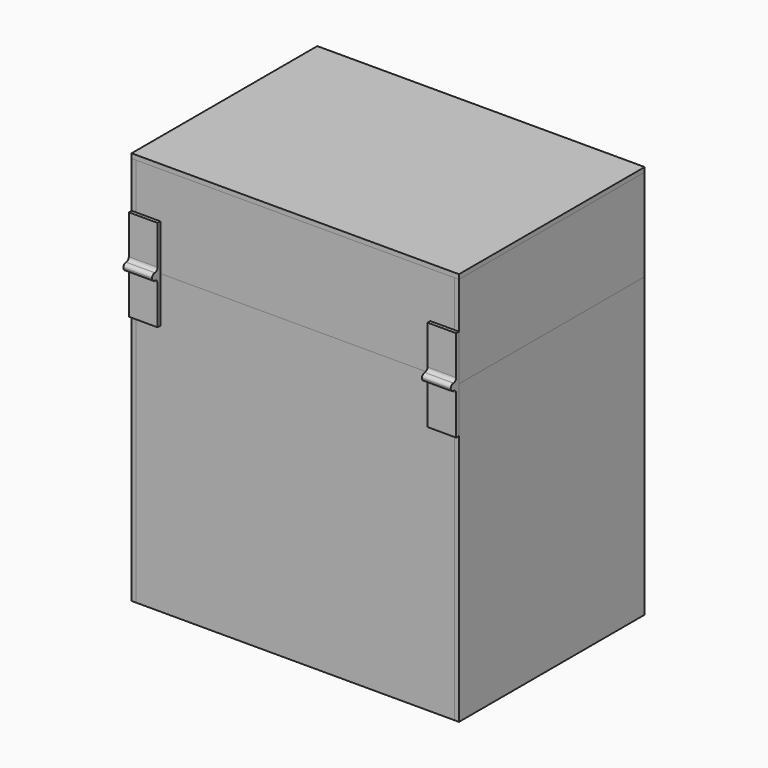
from build123d import *

# Parameters (mm, degrees)
F4_W      = 10
F4_H      = 10
F5_DEPTH  = 245
F6_W      = 276.9150262213
F6_H      = 4
F7_DEPTH  = 245
F8_W      = 4
F8_H      = 202
F9_DEPTH  = 245
F8_H_2    = 140
F10_W     = 284.9150262213
F10_H     = 202
F11_DEPTH = 4
F12_DEPTH = 80
F15_W     = 276.9150262213
F15_H     = 4
F17_DEPTH = 80
F16_W     = 4
F16_H     = 202
F19_W     = 284.9150262213
F19_H     = 202
F20_DEPTH = 4
F24_W     = 4
F24_H     = 194
F25_DEPTH = 40
F24_W_2   = 100
F24_H_2   = 100
F26_W     = 144
F26_H     = 194
F27_DEPTH = 4
F29_W     = 131.9150262213
F29_H     = 192
F30_DEPTH = 4
F32_W     = 114.9150262213
F32_H     = 10
F33_DEPTH = 10
F32_W_2   = 75
F32_W_3   = 10
F32_H_2   = 75
F34_R     = 47.5
F35_DEPTH = 40
F37_DEPTH = 25
F43_W     = 276.9150262213
F43_H     = 4
F44_DEPTH = 14
F45_W     = 4
F45_H     = 202
F46_DEPTH = 14


with BuildPart() as f5:
    # F4 (on Top) → F5 (new body)
    with BuildSketch(Plane.XY):
        with Locations((-139, 135)):
            Rectangle(F4_W, F4_H)
    extrude(amount=F5_DEPTH)


with BuildPart() as f5b:
    # F4 (on Top) → F5, piece 2 (new body)
    with BuildSketch(Plane.XY):
        with Locations((-9, 135)):
            Rectangle(F4_W, F4_H)
    extrude(amount=F5_DEPTH)


with BuildPart() as f5c:
    # F4 (on Top) → F5, piece 3 (new body)
    with BuildSketch(Plane.XY):
        with Locations((5, 135)):
            Rectangle(F4_W, F4_H)
    extrude(amount=F5_DEPTH)


with BuildPart() as f5d:
    # F4 (on Top) → F5, piece 4 (new body)
    with BuildSketch(Plane.XY):
        with Locations((127.9150262213, 135)):
            Rectangle(F4_W, F4_H)
    extrude(amount=F5_DEPTH)


with BuildPart() as f5e:
    # F4 (on Top) → F5, piece 5 (new body)
    with BuildSketch(Plane.XY):
        with Locations((127.9150262213, 5)):
            Rectangle(F4_W, F4_H)
    extrude(amount=F5_DEPTH)


with BuildPart() as f5f:
    # F4 (on Top) → F5, piece 6 (new body)
    with BuildSketch(Plane.XY):
        with Locations((127.9150262213, -49)):
            Rectangle(F4_W, F4_H)
    extrude(amount=F5_DEPTH)


with BuildPart() as f5g:
    # F4 (on Top) → F5, piece 7 (new body)
    with BuildSketch(Plane.XY):
        with Locations((5, 5)):
            Rectangle(F4_W, F4_H)
    extrude(amount=F5_DEPTH)


with BuildPart() as f5h:
    # F4 (on Top) → F5, piece 8 (new body)
    with BuildSketch(Plane.XY):
        with Locations((-9, 5)):
            Rectangle(F4_W, F4_H)
    extrude(amount=F5_DEPTH)


with BuildPart() as f5i:
    # F4 (on Top) → F5, piece 9 (new body)
    with BuildSketch(Plane.XY):
        with Locations((-139, 5)):
            Rectangle(F4_W, F4_H)
    extrude(amount=F5_DEPTH)


with BuildPart() as f5j:
    # F4 (on Top) → F5, piece 10 (new body)
    with BuildSketch(Plane.XY):
        with Locations((-139, -49)):
            Rectangle(F4_W, F4_H)
    extrude(amount=F5_DEPTH)


with BuildPart() as f7:
    # F6 (on Top) → F7 (new body)
    with BuildSketch(Plane.XY):
        with Locations((-5.5424868894, 142)):
            Rectangle(F6_W, F6_H)
    extrude(amount=F7_DEPTH)

    # F43 (on face) → F44, piece 2 (join)
    with BuildSketch(Plane(origin=(0, 0, 0), x_dir=(1, 0, 0), z_dir=(0, 0, -1))):
        with Locations((-5.5424868894, -142)):
            Rectangle(F43_W, F43_H)
    extrude(amount=F44_DEPTH)


with BuildPart() as f7b:
    # F6 (on Top) → F7, piece 2 (new body)
    with BuildSketch(Plane.XY):
        with Locations((-5.5424868894, -2)):
            Rectangle(F6_W, F6_H)
    extrude(amount=F7_DEPTH)


with BuildPart() as f7c:
    # F6 (on Top) → F7, piece 3 (new body)
    with BuildSketch(Plane.XY):
        with Locations((-5.5424868894, -56)):
            Rectangle(F6_W, F6_H)
    extrude(amount=F7_DEPTH)

    # F43 (on face) → F44 (join)
    with BuildSketch(Plane(origin=(0, 0, 0), x_dir=(1, 0, 0), z_dir=(0, 0, -1))):
        with Locations((-5.5424868894, 56)):
            Rectangle(F43_W, F43_H)
    extrude(amount=F44_DEPTH)


with BuildPart() as f9:
    # F8 (on Top) → F9 (new body)
    with BuildSketch(Plane.XY):
        with Locations((-146, 43)):
            Rectangle(F8_W, F8_H)
    extrude(amount=F9_DEPTH)

    # F45 (on face) → F46 (join)
    with BuildSketch(Plane(origin=(0, 0, 0), x_dir=(1, 0, 0), z_dir=(0, 0, -1))):
        with Locations((-146, -43)):
            Rectangle(F45_W, F45_H)
    extrude(amount=F46_DEPTH)


with BuildPart() as f9b:
    # F8 (on Top) → F9, piece 2 (new body)
    with BuildSketch(Plane.XY):
        with Locations((-2, 70)):
            Rectangle(F8_W, F8_H_2)
    extrude(amount=F9_DEPTH)


with BuildPart() as f9c:
    # F8 (on Top) → F9, piece 3 (new body)
    with BuildSketch(Plane.XY):
        with Locations((134.9150262213, 43)):
            Rectangle(F8_W, F8_H)
    extrude(amount=F9_DEPTH)

    # F45 (on face) → F46, piece 2 (join)
    with BuildSketch(Plane(origin=(0, 0, 0), x_dir=(1, 0, 0), z_dir=(0, 0, -1))):
        with Locations((134.9150262213, -43)):
            Rectangle(F45_W, F45_H)
    extrude(amount=F46_DEPTH)


with BuildPart() as f11:
    # F10 (on Top) → F11 (new body)
    with BuildSketch(Plane.XY):
        with Locations((-5.5424868894, 43)):
            Rectangle(F10_W, F10_H)
    extrude(amount=-F11_DEPTH)

    # F47: cut F9c, F7c, F7, F9
    add(f9c.part, mode=Mode.SUBTRACT)
    add(f7c.part, mode=Mode.SUBTRACT)
    add(f7.part, mode=Mode.SUBTRACT)
    add(f9.part, mode=Mode.SUBTRACT)


with BuildPart() as f12:
    # F4 (on Top) → F12 (new body)
    with BuildSketch(Plane.XY):
        with Locations((-139, 135)):
            Rectangle(F4_W, F4_H)
    extrude(amount=F12_DEPTH)


with BuildPart() as f12b:
    # F4 (on Top) → F12, piece 2 (new body)
    with BuildSketch(Plane.XY):
        with Locations((-9, 135)):
            Rectangle(F4_W, F4_H)
    extrude(amount=F12_DEPTH)


with BuildPart() as f12c:
    # F4 (on Top) → F12, piece 3 (new body)
    with BuildSketch(Plane.XY):
        with Locations((5, 135)):
            Rectangle(F4_W, F4_H)
    extrude(amount=F12_DEPTH)


with BuildPart() as f12d:
    # F4 (on Top) → F12, piece 4 (new body)
    with BuildSketch(Plane.XY):
        with Locations((127.9150262213, 135)):
            Rectangle(F4_W, F4_H)
    extrude(amount=F12_DEPTH)


with BuildPart() as f12e:
    # F4 (on Top) → F12, piece 5 (new body)
    with BuildSketch(Plane.XY):
        with Locations((127.9150262213, 5)):
            Rectangle(F4_W, F4_H)
    extrude(amount=F12_DEPTH)


with BuildPart() as f12f:
    # F4 (on Top) → F12, piece 6 (new body)
    with BuildSketch(Plane.XY):
        with Locations((127.9150262213, -49)):
            Rectangle(F4_W, F4_H)
    extrude(amount=F12_DEPTH)


with BuildPart() as f12g:
    # F4 (on Top) → F12, piece 7 (new body)
    with BuildSketch(Plane.XY):
        with Locations((5, 5)):
            Rectangle(F4_W, F4_H)
    extrude(amount=F12_DEPTH)


with BuildPart() as f12h:
    # F4 (on Top) → F12, piece 8 (new body)
    with BuildSketch(Plane.XY):
        with Locations((-9, 5)):
            Rectangle(F4_W, F4_H)
    extrude(amount=F12_DEPTH)


with BuildPart() as f12i:
    # F4 (on Top) → F12, piece 9 (new body)
    with BuildSketch(Plane.XY):
        with Locations((-139, 5)):
            Rectangle(F4_W, F4_H)
    extrude(amount=F12_DEPTH)


with BuildPart() as f12j:
    # F4 (on Top) → F12, piece 10 (new body)
    with BuildSketch(Plane.XY):
        with Locations((-139, -49)):
            Rectangle(F4_W, F4_H)
    extrude(amount=F12_DEPTH)


with BuildPart() as f12j_1:
    # F13: moved
    add(f12j.part.moved(Location((0, 0, 245))))


with BuildPart() as f12i_1:
    # F13: moved
    add(f12i.part.moved(Location((0, 0, 245))))


with BuildPart() as f12h_1:
    # F13: moved
    add(f12h.part.moved(Location((0, 0, 245))))


with BuildPart() as f12g_1:
    # F13: moved
    add(f12g.part.moved(Location((0, 0, 245))))


with BuildPart() as f12f_1:
    # F13: moved
    add(f12f.part.moved(Location((0, 0, 245))))


with BuildPart() as f12e_1:
    # F13: moved
    add(f12e.part.moved(Location((0, 0, 245))))


with BuildPart() as f12d_1:
    # F13: moved
    add(f12d.part.moved(Location((0, 0, 245))))


with BuildPart() as f12c_1:
    # F13: moved
    add(f12c.part.moved(Location((0, 0, 245))))


with BuildPart() as f12b_1:
    # F13: moved
    add(f12b.part.moved(Location((0, 0, 245))))


with BuildPart() as f12_1:
    # F13: moved
    add(f12.part.moved(Location((0, 0, 245))))


with BuildPart() as f17:
    # F15 (on offset) → F17 (new body)
    with BuildSketch(Plane.XY.offset(245)):
        with Locations((-5.5424868894, -56)):
            Rectangle(F15_W, F15_H)
    extrude(amount=F17_DEPTH)


with BuildPart() as f17b:
    # F15 (on offset) → F17, piece 2 (new body)
    with BuildSketch(Plane.XY.offset(245)):
        with Locations((-5.5424868894, 142)):
            Rectangle(F15_W, F15_H)
    extrude(amount=F17_DEPTH)


with BuildPart() as f17c:
    # F16 (on offset) → F17, piece 3 (new body)
    with BuildSketch(Plane.XY.offset(245)):
        with Locations((-146, 43)):
            Rectangle(F16_W, F16_H)
    extrude(amount=F17_DEPTH)


with BuildPart() as f17d:
    # F16 (on offset) → F17, piece 4 (new body)
    with BuildSketch(Plane.XY.offset(245)):
        with Locations((134.9150262213, 43)):
            Rectangle(F16_W, F16_H)
    extrude(amount=F17_DEPTH)


with BuildPart() as f20:
    # F19 (on offset) → F20 (new body)
    with BuildSketch(Plane.XY.offset(325)):
        with Locations((-5.5424868894, 43)):
            Rectangle(F19_W, F19_H)
    extrude(amount=F20_DEPTH)


with BuildPart() as f23_1:
    # F23: copy of F12b
    add(f12b_1.part.moved(Location((0, -184, 0))))


with BuildPart() as f23_2:
    # F23: copy of F12c
    add(f12c_1.part.moved(Location((0, -184, 0))))


with BuildPart() as f25:
    # F24 (on offset) → F25 (new body)
    with BuildSketch(Plane.XY.offset(245)):
        with Locations((-2, 43)):
            Rectangle(F24_W, F24_H)
    extrude(amount=F25_DEPTH)


with BuildPart() as f25b:
    # F24 (on offset) → F25, piece 2 (new body)
    with BuildSketch(Plane.XY.offset(245)):
        with Locations((-74, 70)):
            Rectangle(F24_W_2, F24_H_2)
    extrude(amount=F25_DEPTH)


with BuildPart() as f27:
    # F26 (on offset) → F27 (new body)
    with BuildSketch(Plane.XY.offset(245)):
        with Locations((-72, 43)):
            Rectangle(F26_W, F26_H)
    extrude(amount=F27_DEPTH)


with BuildPart() as f25_1:
    add(f25.part)

    # F28: cut F27
    add(f27.part, mode=Mode.SUBTRACT)


with BuildPart() as f12j_2:
    add(f12j_1.part)

    # F28: cut F27
    add(f27.part, mode=Mode.SUBTRACT)


with BuildPart() as f23_1_1:
    add(f23_1.part)

    # F28: cut F27
    add(f27.part, mode=Mode.SUBTRACT)


with BuildPart() as f12_2:
    add(f12_1.part)

    # F28: cut F27
    add(f27.part, mode=Mode.SUBTRACT)


with BuildPart() as f12b_2:
    add(f12b_1.part)

    # F28: cut F27
    add(f27.part, mode=Mode.SUBTRACT)


with BuildPart() as f25b_1:
    add(f25b.part)

    # F28: cut F27
    add(f27.part, mode=Mode.SUBTRACT)


with BuildPart() as f30:
    # F29 (on offset) → F30 (new body)
    with BuildSketch(Plane.XY.offset(245)):
        with Locations((65.9575131106, 44)):
            Rectangle(F29_W, F29_H)
    extrude(amount=F30_DEPTH)


with BuildPart() as f12d_2:
    add(f12d_1.part)

    # F31: cut F30
    add(f30.part, mode=Mode.SUBTRACT)


with BuildPart() as f12c_2:
    add(f12c_1.part)

    # F31: cut F30
    add(f30.part, mode=Mode.SUBTRACT)


with BuildPart() as f23_2_1:
    add(f23_2.part)

    # F31: cut F30
    add(f30.part, mode=Mode.SUBTRACT)


with BuildPart() as f12f_2:
    add(f12f_1.part)

    # F31: cut F30
    add(f30.part, mode=Mode.SUBTRACT)


with BuildPart() as f33:
    # F32 (on face) → F33 (new body)
    with BuildSketch(Plane.XY.offset(249)):
        with Locations((66.4575131106, 135)):
            Rectangle(F32_W, F32_H)
    extrude(amount=F33_DEPTH)


with BuildPart() as f33b:
    # F32 (on face) → F33, piece 2 (new body)
    with BuildSketch(Plane.XY.offset(249)):
        with Locations((66.4575131106, -49)):
            Rectangle(F32_W, F32_H)
    extrude(amount=F33_DEPTH)


with BuildPart() as f33c:
    # F32 (on face) → F33, piece 3 (new body)
    with BuildSketch(Plane.XY.offset(249)):
        with Locations((-74, 135)):
            Rectangle(F32_W_2, F32_H)
    extrude(amount=F33_DEPTH)


with BuildPart() as f33d:
    # F32 (on face) → F33, piece 4 (new body)
    with BuildSketch(Plane.XY.offset(249)):
        with Locations((-9, 43)):
            Rectangle(F32_W_3, F32_H_2)
    extrude(amount=F33_DEPTH)


with BuildPart() as f33e:
    # F32 (on face) → F33, piece 5 (new body)
    with BuildSketch(Plane.XY.offset(249)):
        with Locations((5, 43)):
            Rectangle(F32_W_3, F32_H_2)
    extrude(amount=F33_DEPTH)


with BuildPart() as f33f:
    # F32 (on face) → F33, piece 6 (new body)
    with BuildSketch(Plane.XY.offset(249)):
        with Locations((127.9150262213, 43)):
            Rectangle(F32_W_3, F32_H_2)
    extrude(amount=F33_DEPTH)


with BuildPart() as f33g:
    # F32 (on face) → F33, piece 7 (new body)
    with BuildSketch(Plane.XY.offset(249)):
        with Locations((-74, -49)):
            Rectangle(F32_W_2, F32_H)
    extrude(amount=F33_DEPTH)


with BuildPart() as f33h:
    # F32 (on face) → F33, piece 8 (new body)
    with BuildSketch(Plane.XY.offset(249)):
        with Locations((-139, 43)):
            Rectangle(F32_W_3, F32_H_2)
    extrude(amount=F33_DEPTH)


with BuildPart() as f35_tool:
    # F34 (on face) → F35 (new body, symmetric)
    with BuildSketch(Plane.XY.offset(249)):
        with Locations((-74, 70)):
            Circle(F34_R)
    extrude(amount=F35_DEPTH, both=True)


with BuildPart() as f25b_2:
    add(f25b_1.part)

    # F35: cut by f35_tool
    add(f35_tool.part, mode=Mode.SUBTRACT)


with BuildPart() as f27_1:
    add(f27.part)

    # F35: cut by f35_tool
    add(f35_tool.part, mode=Mode.SUBTRACT)


with BuildPart() as f37:
    # F36 (on face) → F37 (new body)
    with BuildSketch(Plane.YZ.offset(136.9150262213)):
        with BuildLine():
            Line((-58, 245), (-58, 285))
            Line((-58, 285), (-61, 285))
            Line((-61, 285), (-61, 251))
            ThreePointArc((-61, 251), (-61.8786796564, 248.8786796564), (-64, 248))
            ThreePointArc((-64, 248), (-66.1213203436, 247.1213203436), (-67, 245))
            ThreePointArc((-67, 245), (-66.1213203436, 242.8786796564), (-64, 242))
            ThreePointArc((-64, 242), (-61.8786796564, 241.1213203436), (-61, 239))
            Line((-61, 239), (-61, 205))
            Line((-61, 205), (-58, 205))
            Line((-58, 205), (-58, 245))
        make_face()
    extrude(amount=-F37_DEPTH)


with BuildPart() as f38_1:
    # F38: copy of F37
    add(f37.part.moved(Location((-284.9150262213, 0, 0))))


with BuildPart() as f38_1_1:
    # F39: moved
    add(f38_1.part.moved(Location((25, 0, 0))))


with BuildPart() as f40_1:
    # F40: copy of F33
    add(f33.part.moved(Location((0, 0, 66))))


with BuildPart() as f40_2:
    # F40: copy of F33b
    add(f33b.part.moved(Location((0, 0, 66))))


with BuildPart() as f40_3:
    # F40: copy of F33c
    add(f33c.part.moved(Location((0, 0, 66))))


with BuildPart() as f40_4:
    # F40: copy of F33d
    add(f33d.part.moved(Location((0, 0, 66))))


with BuildPart() as f40_5:
    # F40: copy of F33e
    add(f33e.part.moved(Location((0, 0, 66))))


with BuildPart() as f40_6:
    # F40: copy of F33f
    add(f33f.part.moved(Location((0, 0, 66))))


with BuildPart() as f40_7:
    # F40: copy of F33g
    add(f33g.part.moved(Location((0, 0, 66))))


with BuildPart() as f40_8:
    # F40: copy of F33h
    add(f33h.part.moved(Location((0, 0, 66))))


with BuildPart() as f41_1:
    # F41: copy of F12j
    add(f12j_2.part.moved(Location((10, 0, 0))))


with BuildPart() as f42_1:
    # F42: copy of F12f
    add(f12f_2.part.moved(Location((-10, 0, 0))))


solid = Compound([f5.part, f5b.part, f5c.part, f5d.part, f5e.part, f5f.part, f5g.part, f5h.part, f5i.part, f5j.part, f7.part, f7b.part, f7c.part, f9.part, f9b.part, f9c.part, f11.part, f17.part, f17b.part, f17c.part, f17d.part, f20.part, f25_1.part, f12j_2.part, f23_1_1.part, f12_2.part, f12b_2.part, f30.part, f12d_2.part, f12c_2.part, f23_2_1.part, f12f_2.part, f33.part, f33b.part, f33c.part, f33d.part, f33e.part, f33f.part, f33g.part, f33h.part, f25b_2.part, f27_1.part, f37.part, f38_1_1.part, f40_1.part, f40_2.part, f40_3.part, f40_4.part, f40_5.part, f40_6.part, f40_7.part, f40_8.part, f41_1.part, f42_1.part])
